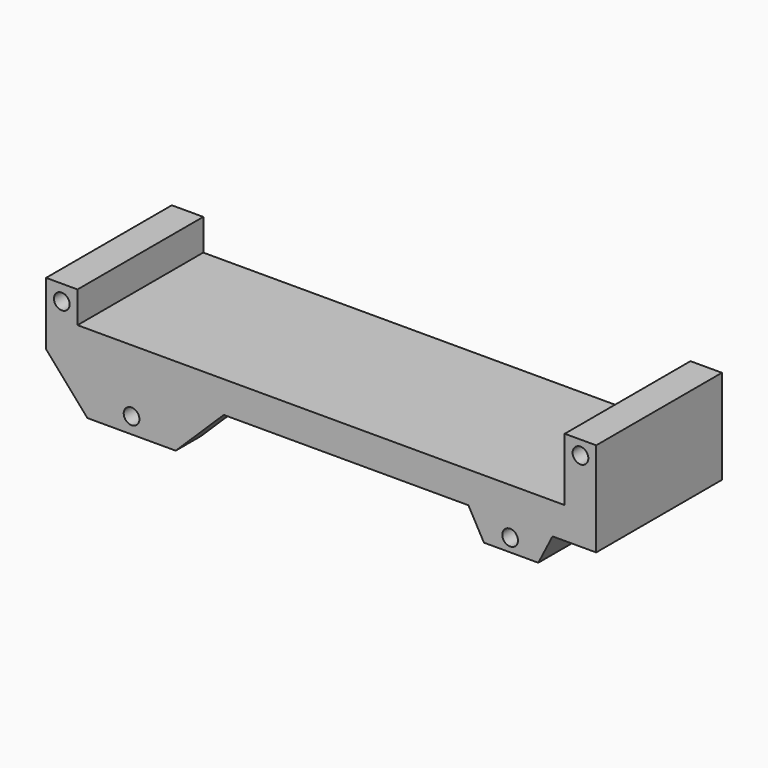
from build123d import *

# Parameters (mm, degrees)
F0_W     = 20
F0_H     = 20
F0_R     = 5
F0_H_2   = 40
F1_DEPTH = 100
F2_W     = 60
F2_H     = 34.6079095881
F3_DEPTH = 131.6404025087


# Not quite as in the source:
# - a feature names something its author has since deleted; it is built from what else it names


with BuildPart() as f1:
    # F0 (on Front) → F1 (new body)
    with BuildSketch(Plane.XZ):
        Polygon((-131.6394025087, 20), (-131.6394025087, 0), (-18.5843738595, 0), (137.0734572411, 0), (190.578520298, 0), (218.3605974913, 0), (218.3605974913, 20), (198.3605974913, 20), (-111.6394025087, 20), align=None)
        with Locations((-121.6394025087, 30)):
            Rectangle(F0_W, F0_H)
        with Locations((-121.6394025087, 30)):
            Circle(F0_R, mode=Mode.SUBTRACT)
        with Locations((208.3605974913, 40)):
            Rectangle(F0_W, F0_H_2)
        with Locations((208.3605974913, 51.0531589389)):
            Circle(F0_R, mode=Mode.SUBTRACT)
        Polygon((190.578520298, 0), (137.0734572411, 0), (146.9386657926, -17.7425388247), (181.5354246128, -17.7425388247), align=None)
        with Locations((163.6041871454, -9.4907971493)):
            Circle(F0_R, mode=Mode.SUBTRACT)
        Polygon((-18.5843738595, 0), (-131.6394025087, 0), (-105.3372249007, -30), (-49.1586900184, -30), align=None)
        with Locations((-77.2479574596, -19.8998747039)):
            Circle(F0_R, mode=Mode.SUBTRACT)
    extrude(amount=F1_DEPTH)

    # F2 (on Right) → F3 (cut, through all)
    with BuildSketch(Plane.YZ):
        with Locations((-50, -17.3039547941)):
            Rectangle(F2_W, F2_H)
    extrude(amount=-F3_DEPTH, mode=Mode.SUBTRACT)


solid = f1.part
